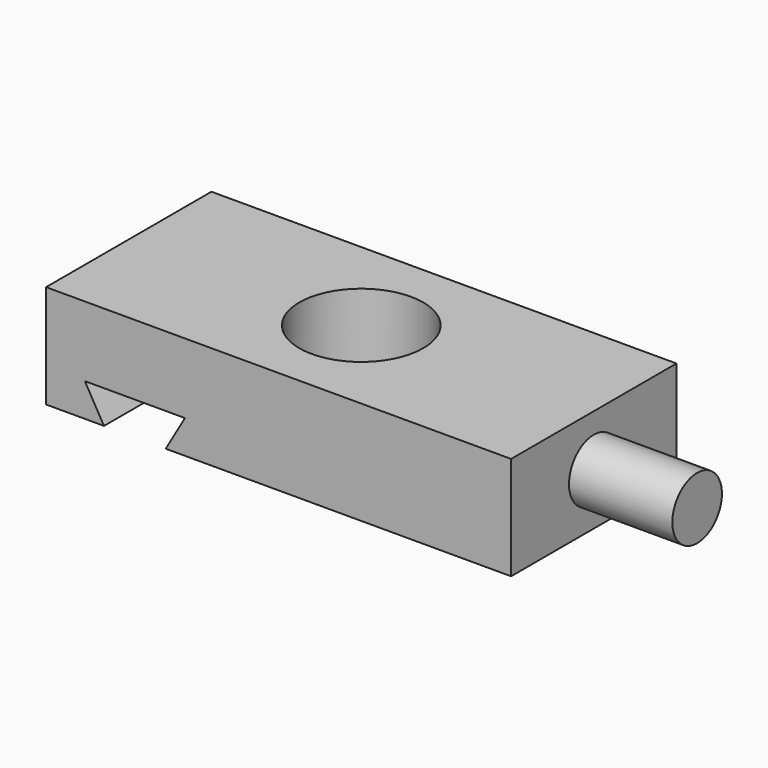
from build123d import *

# Parameters (mm, degrees)
F0_W     = 114.3
F0_H     = 50.8
F0_R     = 15.24
F1_DEPTH = 25.4
F4_DEPTH = 50.801
F5_R     = 7.62
F6_DEPTH = 25.4


# Not quite as in the source:
# - ends of sketch curves that miss each other by under 0.0002 mm in the source are joined


with BuildPart() as f1:
    # F0 (on Top) → F1 (new body)
    with BuildSketch(Plane.XY):
        Rectangle(F0_W, F0_H)
        Circle(F0_R, mode=Mode.SUBTRACT)
    extrude(amount=F1_DEPTH)

    # F3 (on face) → F4 (cut, through all)
    with BuildSketch(Plane(origin=(0, 25.4, 0), x_dir=(-1, 0, 0), z_dir=(0, 1, 0))):
        Polygon((27.7357548475, 0), (42.9095774889, 0), (47.6239210906, 8.1654826425), (23.0214107298, 8.1654835362), align=None)
    extrude(amount=-F4_DEPTH, mode=Mode.SUBTRACT)

    # F5 (on face) → F6 (join)
    with BuildSketch(Plane.YZ.offset(57.15)):
        with Locations((0, 12.7)):
            Circle(F5_R)
    extrude(amount=F6_DEPTH)


solid = f1.part
